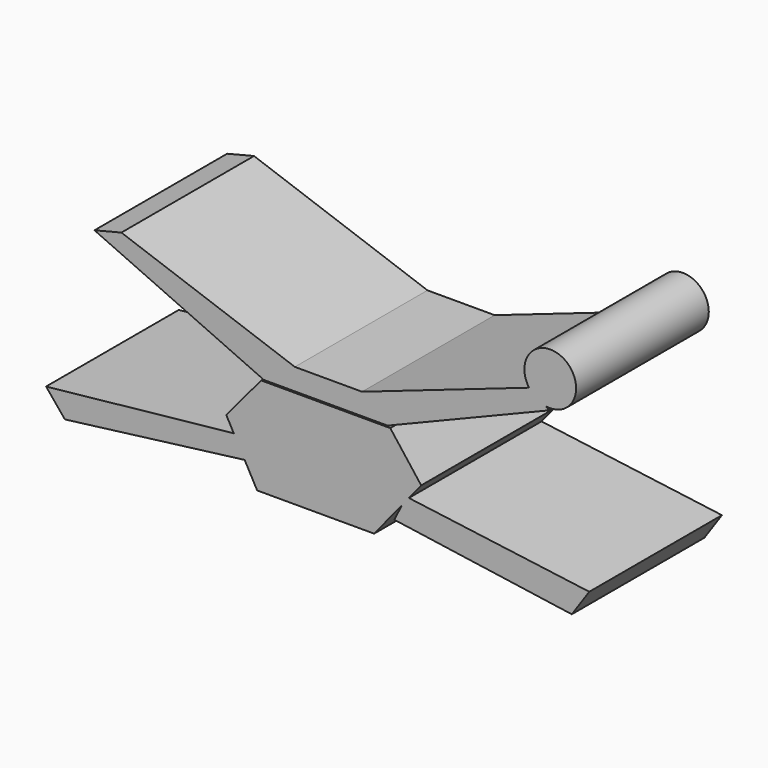
from build123d import *

# Parameters (mm, degrees)
F2_R      = 3.9614488342
F3_DEPTH  = 25.4
F5_DEPTH  = 25.4
F7_DEPTH  = 25.4
F9_DEPTH  = 25.4
F11_DEPTH = 25.4


# Not quite as in the source:
# - the program builds the solid bodies; features that only make, move or delete a surface that nothing else refers to are left out


with BuildPart() as f3:
    # F2 (on Front) → F3 (new body)
    with BuildSketch(Plane.XZ):
        with Locations((33.2602709532, 23.0659469962)):
            Circle(F2_R)
    extrude(amount=F3_DEPTH)

    # F4 (on Front) → F5 (join)
    with BuildSketch(Plane.XZ):
        Polygon((-5.8694598265, 11.9448658079), (-32.4364863336, 21.4183777571), (-36.5554057062, 20.3886479139), (-10.6062162668, 8.6497301236), (8.3408113569, 8.6497301236), (33.0543257296, 18.7410805374), (30.5829718709, 21.0064873099), (4.4278376736, 11.9448658079), align=None)
    extrude(amount=F5_DEPTH)


with BuildPart() as f7:
    # F6 (on Front) → F7 (new body)
    with BuildSketch(Plane.XZ):
        Polygon((8.7527008727, 8.4437839687), (-11.0181085765, 8.4437839687), (-16.3727030158, 2.0594594534), (-11.6359470412, -6.5902704373), (6.2813521363, -6.5902704373), (13.4894605726, 2.2654053755), align=None)
    extrude(amount=F7_DEPTH)

    # F8 (on Front) → F9 (join)
    with BuildSketch(Plane.XZ):
        Polygon((-13.4894596413, -3.0891890638), (-14.7251356393, 0), (-43.9694598317, -3.0891890638), (-41.0862155259, -6.5902704373), align=None)
    extrude(amount=F9_DEPTH)

    # F10 (on Front) → F11 (join)
    with BuildSketch(Plane.XZ):
        Polygon((39.2327047884, -3.7070270628), (11.2240547314, 0), (9.3705402687, -3.7070270628), (36.5554057062, -7.6200002804), align=None)
    extrude(amount=F11_DEPTH)


solid = Compound([f3.part, f7.part])
